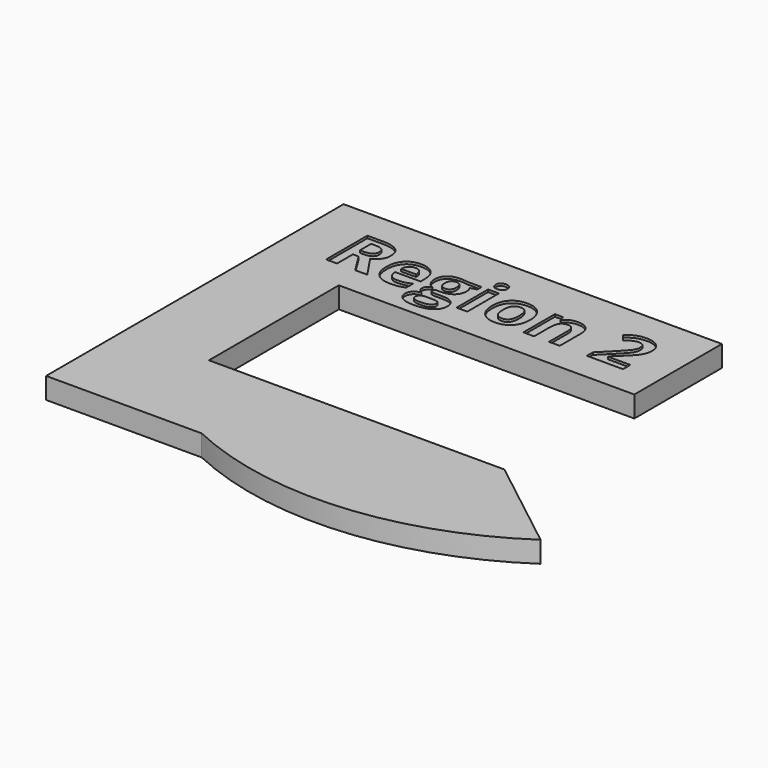
from build123d import *

# Parameters (mm, degrees)
F1_DEPTH     = 4.5
F2_TEXT_SIZE = 15.3586009724
F3_DEPTH     = 0.5


# Not quite as in the source:
# - Text() gives the source's letters only with a copy of the font that has no kerning and outlines rounded to 1/6400 em; it was checked with that copy


with BuildPart() as f1:
    # F0 (on Top) → F1 (new body)
    with BuildSketch(Plane.XY):
        with BuildLine():
            Line((27.7171041816, 79), (27.7171041816, 0))
            Line((27.7171041816, 0), (60.7638921879, 0))
            ThreePointArc((60.7638921879, 0), (95.350151466, -6.2922661299), (128.5476840938, 5.2717198318))
            Line((128.5476840938, 5.2717198318), (108.0806031823, 21.2448128462))
            Line((108.0806031823, 21.2448128462), (45.3097596765, 21.2448128462))
            Line((45.3097596765, 21.2448128462), (45.3097596765, 55.7404794693))
            Line((45.3097596765, 55.7404794693), (90, 55.7404794693))
            Line((90, 55.7404794693), (108.0806031823, 55.7404794693))
            Line((108.0806031823, 55.7404794693), (108.0806031823, 79))
            Line((108.0806031823, 79), (27.7171041816, 79))
        make_face()
    extrude(amount=F1_DEPTH)

    # F2 (on face) → F3 (cut)
    with BuildSketch(Plane.XY.offset(4.5)):
        with Locations((36.4758446813, 61.6725198925)):
            Text('Region 2', F2_TEXT_SIZE, font='Open Sans', font_style=FontStyle.BOLD, text_align=(TextAlign.LEFT, TextAlign.BOTTOM))
    extrude(amount=-F3_DEPTH, mode=Mode.SUBTRACT)


solid = f1.part
